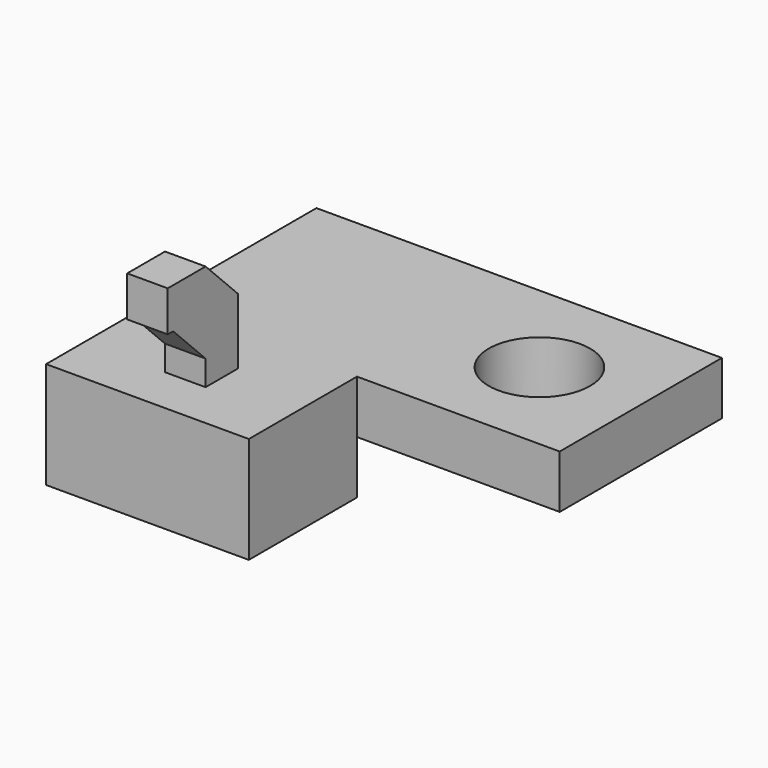
from build123d import *

# Parameters (mm, degrees)
F0_R     = 1.905
F0_W     = 7.62
F0_H     = 5.08
F0_W_2   = 1.524
F0_H_2   = 1.524
F1_DEPTH = 2
F2_DEPTH = 2
F3_DEPTH = 5.9944
F4_W     = 1.524
F4_H     = 1.524
F5_DEPTH = 2.4638
F6_SIZE  = 1.524


# Not quite as in the source:
# - a feature names something its author has since deleted; it is built from what else it names


with BuildPart() as f1:
    # F0 (on Top) → F1 (new body)
    with BuildSketch(Plane.XY):
        Polygon((-32.4838893509, -2.5229738411), (-32.4838893509, 5.0970261589), (-47.7238893509, 5.0970261589), (-47.7238893509, -2.5229738411), (-40.1038893509, -2.5229738411), align=None)
        with Locations((-36.2938893509, 1.2870261589)):
            Circle(F0_R, mode=Mode.SUBTRACT)
        with Locations((-43.9138893509, -5.0629738411)):
            Rectangle(F0_W, F0_H)
        with Locations((-43.9138893509, -5.0629738411)):
            Rectangle(F0_W_2, F0_H_2, mode=Mode.SUBTRACT)
    extrude(amount=F1_DEPTH)

    # F0 (on Top) → F2 (join)
    with BuildSketch(Plane.XY):
        with Locations((-43.9138893509, -5.0629738411)):
            Rectangle(F0_W, F0_H)
        with Locations((-43.9138893509, -5.0629738411)):
            Rectangle(F0_W_2, F0_H_2, mode=Mode.SUBTRACT)
    extrude(amount=-F2_DEPTH)

    # F0 (on Top) → F3 (join)
    with BuildSketch(Plane.XY):
        with Locations((-43.9138893509, -5.0629738411)):
            Rectangle(F0_W_2, F0_H_2)
    extrude(amount=F3_DEPTH)

    # F4 (on face) → F5 (join)
    with BuildSketch(Plane.XZ.offset(7.6029738411)):
        with Locations((-43.9138893509, 5.2324)):
            Rectangle(F4_W, F4_H)
    extrude(amount=-F5_DEPTH)

    # F6
    f6_edges = [f1.edges().sort_by_distance(p)[0] for p in [
        (-43.913889, -5.824974, 4.4704),
        (-43.913889, -4.300974, 5.9944),
    ]]
    chamfer(f6_edges, length=F6_SIZE)


solid = f1.part
